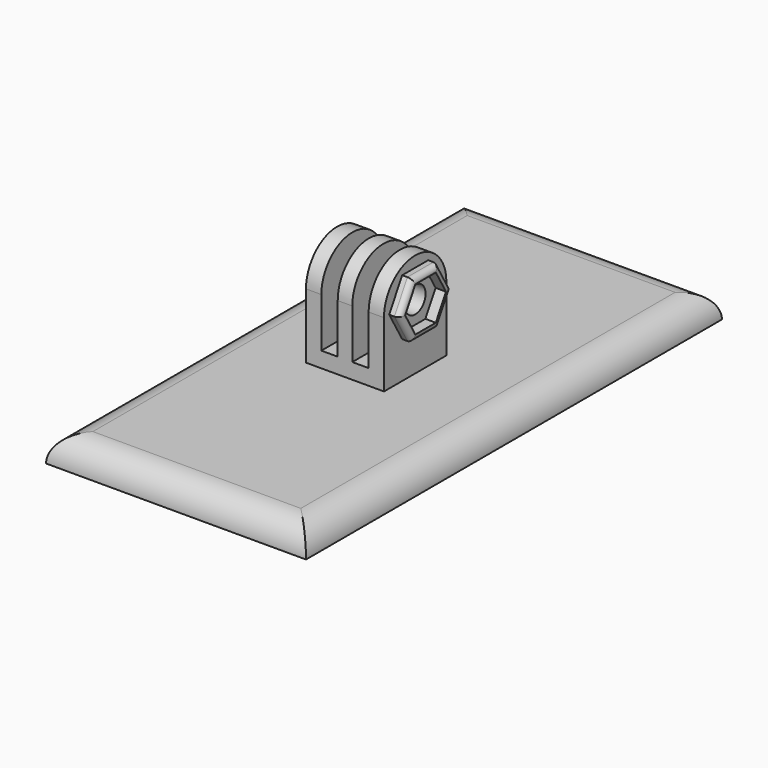
from build123d import *

# Parameters (mm, degrees)
F0_W      = 15
F0_H      = 3
F1_DEPTH  = 15
F2_DEPTH  = 3
F3_DEPTH  = 3
F4_DEPTH  = 2
F5_DEPTH  = 3
F6_DEPTH  = 12
F7_D      = 5
F7_DEPTH  = 15
F7_TIP    = 1.5021515476
F9_W      = 3.15
F9_H      = 15
F10_DEPTH = 17
F11_R     = 1
F12_W     = 50
F12_H     = 100
F13_DEPTH = 5
F14_R     = 4.99999


# Not quite as in the source:
# - a fillet or chamfer is up to 0.001 mm smaller than in the source, because OpenCascade refuses the exact size


with BuildPart() as f1:
    # F0 (on Right) → F1 (new body)
    with BuildSketch(Plane.YZ):
        with Locations((0, 1.5)):
            Rectangle(F0_W, F0_H)
    extrude(amount=-F1_DEPTH)

    # F0 (on Right) → F2 (join)
    with BuildSketch(Plane.YZ):
        with BuildLine():
            Line((-7.5, 12.5), (-7.5, 3))
            Line((-7.5, 3), (7.5, 3))
            Line((7.5, 3), (7.5, 12.5))
            ThreePointArc((7.5, 12.5), (0, 20), (-7.5, 12.5))
        make_face()
        Polygon((-6.25, 12.5), (-3.125, 17.9126587737), (3.125, 17.9126587737), (6.25, 12.5), (3.125, 7.0873412263), (-3.125, 7.0873412263), align=None, mode=Mode.SUBTRACT)
    extrude(amount=-F2_DEPTH)

    # F0 (on Right) → F3 (join)
    with BuildSketch(Plane.YZ):
        Polygon((3.125, 17.9126587737), (-3.125, 17.9126587737), (-6.25, 12.5), (-3.125, 7.0873412263), (3.125, 7.0873412263), (6.25, 12.5), align=None)
        Polygon((-4.9074772881, 12.5), (-2.4537386441, 16.75), (2.4537386441, 16.75), (4.9074772881, 12.5), (2.4537386441, 8.25), (-2.4537386441, 8.25), align=None, mode=Mode.SUBTRACT)
    extrude(amount=-F3_DEPTH)

    # F0 (on Right) → F4 (join)
    with BuildSketch(Plane.YZ):
        Polygon((3.125, 17.9126587737), (-3.125, 17.9126587737), (-6.25, 12.5), (-3.125, 7.0873412263), (3.125, 7.0873412263), (6.25, 12.5), align=None)
        Polygon((-4.9074772881, 12.5), (-2.4537386441, 16.75), (2.4537386441, 16.75), (4.9074772881, 12.5), (2.4537386441, 8.25), (-2.4537386441, 8.25), align=None, mode=Mode.SUBTRACT)
    extrude(amount=F4_DEPTH)

    # F0 (on Right) → F5 (join)
    with BuildSketch(Plane.YZ):
        Polygon((2.4537386441, 16.75), (-2.4537386441, 16.75), (-4.9074772881, 12.5), (-2.4537386441, 8.25), (2.4537386441, 8.25), (4.9074772881, 12.5), align=None)
    extrude(amount=-F5_DEPTH)

    # F6 (add): a face of the model
    f6_faces = [f1.faces().sort_by_distance(p)[0] for p in [
        (-3, 0, 10.7862789639),
    ]]
    extrude(f6_faces, amount=F6_DEPTH)

    # F7
    with Locations(Plane.YZ):
        with Locations((0, 12.5)):
            Hole(F7_D / 2, depth=F7_DEPTH)
            with Locations((0, 0, -(F7_DEPTH + F7_TIP / 2))):  # 118° drill point
                Cone(0, F7_D / 2, F7_TIP, mode=Mode.SUBTRACT)

    # F9 (on offset) → F10 (cut)
    with BuildSketch(Plane.XY.offset(20)):
        with Locations((-10.475, 0)):
            Rectangle(F9_W, F9_H)
        with Locations((-4.525, 0)):
            Rectangle(F9_W, F9_H)
    extrude(amount=-F10_DEPTH, mode=Mode.SUBTRACT)

    # F11
    f11_edges = [f1.edges().sort_by_distance(p)[0] for p in [
        (2, -4.6875, 9.793671),
        (2, 0, 7.087341),
        (2, -4.6875, 15.206329),
        (2, 0, 17.912659),
        (2, 4.6875, 15.206329),
        (2, 4.6875, 9.793671),
    ]]
    fillet(f11_edges, radius=F11_R)

    # F12 (on Top) → F13 (join)
    with BuildSketch(Plane.XY):
        with Locations((-5.9974378107, 0)):
            Rectangle(F12_W, F12_H)
    extrude(amount=-F13_DEPTH)

    # F14 (radius 5 in the source; OpenCascade refuses exactly that, so slightly less here)
    f14_edges = [f1.edges().sort_by_distance(p)[0] for p in [
        (-5.997438, 50, 0),
        (19.002562, 0, 0),
        (-5.997438, -50, 0),
        (-30.997438, 0, 0),
    ]]
    fillet(f14_edges, radius=F14_R)


solid = f1.part
